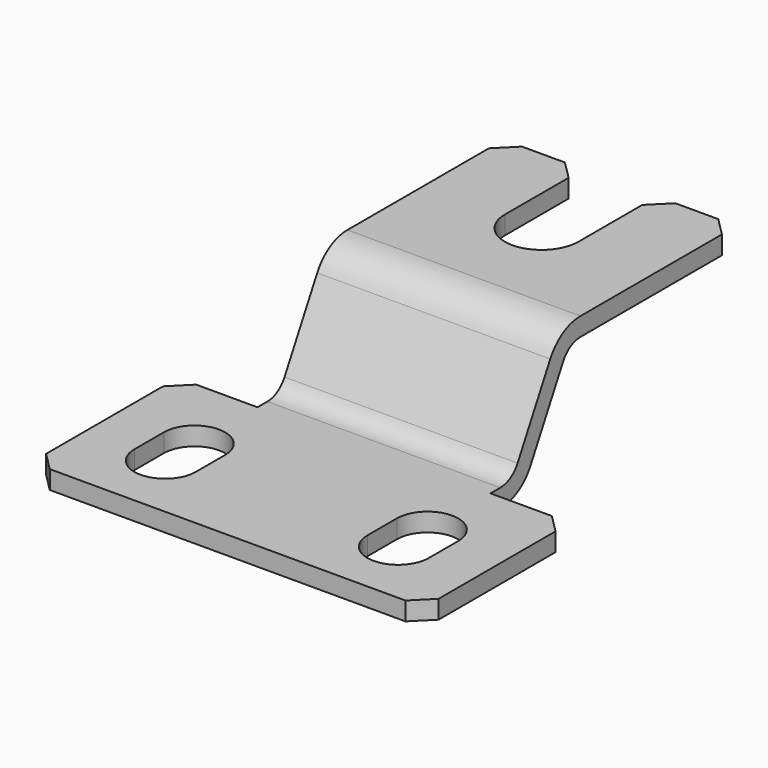
from build123d import *

# Parameters (mm, degrees)
F1_DEPTH = 50.8
F2_R     = 11.1125
F3_W     = 20.6375
F3_H     = 29.0905938273
F3_H_2   = 50.5422030863
F4_DEPTH = 33.3385
F5_SIZE  = 4.7625


with BuildPart() as f1:
    # F0 (on Right) → F1 (new body, symmetric)
    with BuildSketch(Plane.YZ):
        with BuildLine():
            Line((-63.5, 4.7625), (-63.5, 0))
            Line((-63.5, 0), (-6.35, 0))
            Line((-6.35, 0), (7.3786968916, 25.2575142941))
            ThreePointArc((7.3786968916, 25.2575142941), (9.7123359116, 27.6829742473), (12.9577969137, 28.575))
            Line((12.9577969137, 28.575), (63.5, 28.575))
            Line((63.5, 28.575), (63.5, 33.3375))
            Line((63.5, 33.3375), (6.35, 33.3375))
            Line((6.35, 33.3375), (-7.3786968916, 8.0799857059))
            ThreePointArc((-7.3786968916, 8.0799857059), (-9.7123359116, 5.6545257527), (-12.9577969137, 4.7625))
            Line((-12.9577969137, 4.7625), (-63.5, 4.7625))
        make_face()
    extrude(amount=F1_DEPTH, both=True)

    # F2
    f2_edges = [f1.edges().sort_by_distance(p)[0] for p in [
        (0, 6.35, 33.3375),
        (0, -6.35, 0),
    ]]
    fillet(f2_edges, radius=F2_R)

    # F3 (on face) → F4 (cut, through all)
    with BuildSketch(Plane.XY.offset(33.3375)):
        with BuildLine():
            Line((-38.1, -36.5125), (-38.1, -46.0375))
            ThreePointArc((-38.1, -46.0375), (-30.1625, -53.975), (-22.225, -46.0375))
            Line((-22.225, -46.0375), (-22.225, -36.5125))
            ThreePointArc((-22.225, -36.5125), (-30.1625, -28.575), (-38.1, -36.5125))
        make_face()
        with BuildLine():
            ThreePointArc((38.1, -36.5125), (30.1625, -28.575), (22.225, -36.5125))
            Line((22.225, -36.5125), (22.225, -46.0375))
            ThreePointArc((22.225, -46.0375), (30.1625, -53.975), (38.1, -46.0375))
            Line((38.1, -46.0375), (38.1, -36.5125))
        make_face()
        with Locations((-40.48125, -1.5875)):
            Rectangle(F3_W, F3_H)
        with Locations((40.48125, -1.5875)):
            Rectangle(F3_W, F3_H)
        with BuildLine():
            ThreePointArc((9.525, 38.1), (0, 47.625), (-9.525, 38.1))
            ThreePointArc((-9.525, 38.1), (0, 28.575), (9.525, 38.1))
        make_face()
        with BuildLine():
            Line((9.525, 63.5), (-9.525, 63.5))
            Line((-9.525, 63.5), (-9.525, 38.1))
            ThreePointArc((-9.525, 38.1), (0, 47.625), (9.525, 38.1))
            Line((9.525, 38.1), (9.525, 63.5))
        make_face()
        with Locations((-40.48125, 38.2288984568)):
            Rectangle(F3_W, F3_H_2)
        with Locations((40.48125, 38.2288984568)):
            Rectangle(F3_W, F3_H_2)
    extrude(amount=-F4_DEPTH, mode=Mode.SUBTRACT)

    # F5
    f5_edges = [f1.edges().sort_by_distance(p)[0] for p in [
        (50.8, -63.5, 2.38125),
        (50.8, -16.132797, 2.38125),
        (-50.8, -63.5, 2.38125),
        (-50.8, -16.132797, 2.38125),
        (30.1625, 63.5, 30.95625),
        (-30.1625, 63.5, 30.95625),
        (9.525, 63.5, 30.95625),
        (-9.525, 63.5, 30.95625),
    ]]
    chamfer(f5_edges, length=F5_SIZE)


solid = f1.part
